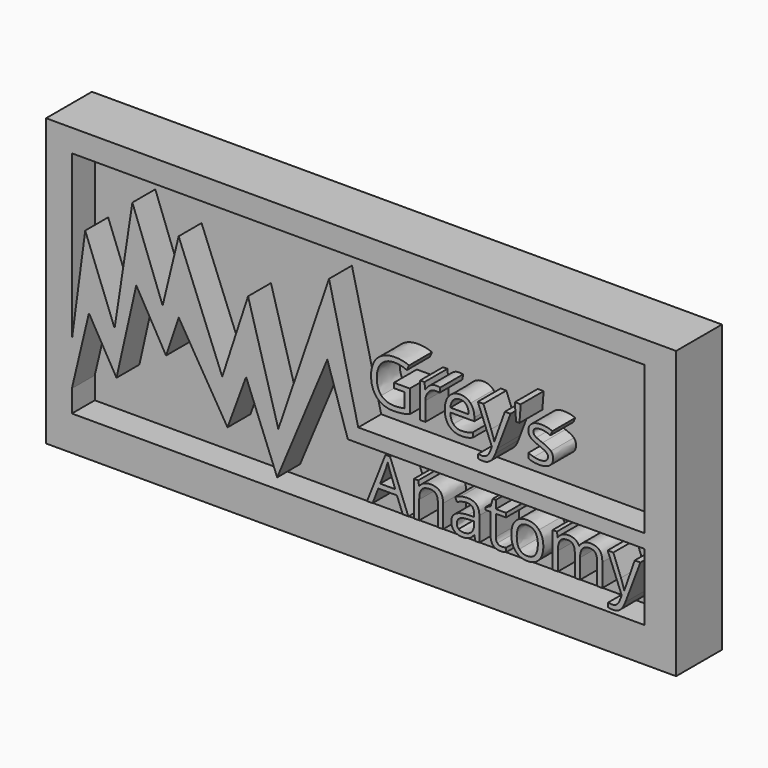
from build123d import *

# Parameters (mm, degrees)
F0_W      = 279.4
F0_H      = 127
F1_DEPTH  = 25.4
F2_DEPTH  = 12.7
F3_DEPTH  = 25.4
F4_DEPTH  = 25.4
F5_DEPTH  = 25.4
F6_DEPTH  = 25.4
F7_DEPTH  = 25.4
F8_DEPTH  = 25.4
F9_DEPTH  = 25.4
F10_DEPTH = 25.4
F11_DEPTH = 25.4
F12_DEPTH = 25.4
F13_DEPTH = 25.4
F14_DEPTH = 25.4
F15_DEPTH = 25.4
F16_DEPTH = 25.4


with BuildPart() as f1:
    # F0 (on Front) → F1 (new body)
    with BuildSketch(Plane.XZ):
        with Locations((-3.9588466167, 0.3931427598)):
            Rectangle(F0_W, F0_H)
        Polygon((-132.2193487672, -18.9143698658), (-132.2193487672, 53.9237214664), (121.7806512328, 53.9237214664), (121.7806512328, 0), (121.7806512328, -11.812004261), (121.7806512328, -17.9444891514), (121.7806512328, -47.6762785336), (-132.2193487672, -47.6762785336), (-132.2193487672, -37.9168875513), align=None, mode=Mode.SUBTRACT)
    extrude(amount=F1_DEPTH)

    # F0 (on Front) → F2 (join)
    with BuildSketch(Plane.XZ):
        Polygon((121.7806512328, 53.9237214664), (-132.2193487672, 53.9237214664), (-132.2193487672, -18.9143698658), (-126.297518611, 25.6726946682), (-113.2765114307, -8.2608237863), (-105.3849980235, 43.4286035597), (-91.969422996, 7.5222076848), (-84.8670601845, 36.9214624689), (-65.5328482389, -11.6113578378), (-54.0901459754, 23.5058874414), (-40.6745709479, -23.958422956), (-18.1837528944, 42.0024342833), (-5.2193487672, -11.812004261), (121.7806512328, -11.812004261), (121.7806512328, 0), align=None)
        with BuildLine():
            Line((24.5695856903, 8.302306513), (24.5695856903, 0))
            Line((24.5695856903, 0), (22.2252456031, 0))
            Line((22.2252456031, 0), (22.2252456031, 15.4708377623))
            Line((22.2252456031, 15.4708377623), (24.1585356943, 15.4708377623))
            Line((24.1585356943, 15.4708377623), (24.4295576697, 12.607038889))
            Line((24.4295576697, 12.607038889), (24.5424834928, 12.607038889))
            add(Edge.make_bspline(
                [(24.5424834928, 12.607038889), (25.4007197482, 14.1157278853), (26.6158016046, 14.9355693609)],
                knots=[0, 0, 0, 1, 1, 1], degree=2))
            add(Edge.make_bspline(
                [(26.6158016046, 14.9355693609), (27.8308834609, 15.7554108365), (29.2853680622, 15.7554108365)],
                knots=[0, 0, 0, 1, 1, 1], degree=2))
            add(Edge.make_bspline(
                [(29.2853680622, 15.7554108365), (30.3152515687, 15.7554108365), (31.1328345279, 15.5837635854)],
                knots=[0, 0, 0, 1, 1, 1], degree=2))
            Line((31.1328345279, 15.5837635854), (30.8076081574, 13.4110707493))
            add(Edge.make_bspline(
                [(30.8076081574, 13.4110707493), (29.8499971776, 13.6233712967), (29.1137208111, 13.6233712967)],
                knots=[0, 0, 0, 1, 1, 1], degree=2))
            add(Edge.make_bspline(
                [(29.1137208111, 13.6233712967), (27.2346351151, 13.6233712967), (25.9021104027, 12.0988726851)],
                knots=[0, 0, 0, 1, 1, 1], degree=2))
            add(Edge.make_bspline(
                [(25.9021104027, 12.0988726851), (24.5695856903, 10.5743740735), (24.5695856903, 8.302306513)],
                knots=[0, 0, 0, 1, 1, 1], degree=2))
        make_face(mode=Mode.SUBTRACT)
        with BuildLine():
            add(Edge.make_bspline(
                [(17.6269060872, 0.7769296628), (16.0347938346, 0.2681554995), (14.391576733, 0)],
                knots=[0, 0, 0, 0.9709878678, 0.9709878678, 0.9709878678], degree=2))
            add(Edge.make_bspline(
                [(14.391576733, 0), (14.3424790734, -0.0080122142), (14.2933357898, -0.0158096152)],
                knots=[0.9709878678, 0.9709878678, 0.9709878678, 1, 1, 1], degree=2))
            add(Edge.make_bspline(
                [(14.2933357898, -0.0158096152), (12.5994484435, -0.2845730742), (10.3680341794, -0.2845730742)],
                knots=[0, 0, 0, 1, 1, 1], degree=2))
            add(Edge.make_bspline(
                [(10.3680341794, -0.2845730742), (8.8718543134, -0.2845730742), (7.5872032589, 0)],
                knots=[0, 0, 0, 0.319412416, 0.319412416, 0.319412416], degree=2))
            add(Edge.make_bspline(
                [(7.5872032589, 0), (4.8499347192, 0.6063537023), (3.0730260083, 2.504694756)],
                knots=[0.319412416, 0.319412416, 0.319412416, 1, 1, 1], degree=2))
            add(Edge.make_bspline(
                [(3.0730260083, 2.504694756), (0.4621809786, 5.2939625861), (0.4621809786, 10.3169031968)],
                knots=[0, 0, 0, 1, 1, 1], degree=2))
            add(Edge.make_bspline(
                [(0.4621809786, 10.3169031968), (0.4621809786, 13.5375476712), (1.7540523947, 15.9586773181)],
                knots=[0, 0, 0, 1, 1, 1], degree=2))
            add(Edge.make_bspline(
                [(1.7540523947, 15.9586773181), (3.0459238107, 18.3798069649), (5.473829007, 19.6558687658)],
                knots=[0, 0, 0, 1, 1, 1], degree=2))
            add(Edge.make_bspline(
                [(5.473829007, 19.6558687658), (7.9017342033, 20.9319305666), (11.158514941, 20.9319305666)],
                knots=[0, 0, 0, 1, 1, 1], degree=2))
            add(Edge.make_bspline(
                [(11.158514941, 20.9319305666), (14.4649830409, 20.9319305666), (17.3152308155, 19.7213657432)],
                knots=[0, 0, 0, 1, 1, 1], degree=2))
            Line((17.3152308155, 19.7213657432), (16.3847220333, 17.6028773021))
            add(Edge.make_bspline(
                [(16.3847220333, 17.6028773021), (13.5886786537, 18.786339928), (11.0049358216, 18.786339928)],
                knots=[0, 0, 0, 1, 1, 1], degree=2))
            add(Edge.make_bspline(
                [(11.0049358216, 18.786339928), (7.2377303636, 18.786339928), (5.1192419225, 16.5436330816)],
                knots=[0, 0, 0, 1, 1, 1], degree=2))
            add(Edge.make_bspline(
                [(5.1192419225, 16.5436330816), (3.0007534815, 14.3009262352), (3.0007534815, 10.3169031968)],
                knots=[0, 0, 0, 1, 1, 1], degree=2))
            add(Edge.make_bspline(
                [(3.0007534815, 10.3169031968), (3.0007534815, 6.1386477428), (5.0401938464, 3.9795060054)],
                knots=[0, 0, 0, 1, 1, 1], degree=2))
            add(Edge.make_bspline(
                [(5.0401938464, 3.9795060054), (7.0796342112, 1.8203642681), (11.0320380191, 1.8203642681)],
                knots=[0, 0, 0, 1, 1, 1], degree=2))
            add(Edge.make_bspline(
                [(11.0320380191, 1.8203642681), (13.1776286577, 1.8203642681), (15.223844572, 2.3172378897)],
                knots=[0, 0, 0, 1, 1, 1], degree=2))
            Line((15.223844572, 2.3172378897), (15.223844572, 8.6681861798))
            Line((15.223844572, 8.6681861798), (10.6119539573, 8.6681861798))
            Line((10.6119539573, 8.6681861798), (10.6119539573, 10.8137768184))
            Line((10.6119539573, 10.8137768184), (17.6269060872, 10.8137768184))
            Line((17.6269060872, 10.8137768184), (17.6269060872, 0.7769296628))
        make_face(mode=Mode.SUBTRACT)
        with BuildLine():
            add(Edge.make_bspline(
                [(45.5873398825, 0.7182082348), (44.4687381201, 0.2382263877), (43.4600252029, 0)],
                knots=[0, 0, 0, 0.9005120931, 0.9005120931, 0.9005120931], degree=2))
            add(Edge.make_bspline(
                [(43.4600252029, 0), (43.3485833493, -0.0263190743), (43.2384827623, -0.0496873622)],
                knots=[0.9005120931, 0.9005120931, 0.9005120931, 1, 1, 1], degree=2))
            add(Edge.make_bspline(
                [(43.2384827623, -0.0496873622), (42.1318096961, -0.2845730742), (40.5643992717, -0.2845730742)],
                knots=[0, 0, 0, 1, 1, 1], degree=2))
            add(Edge.make_bspline(
                [(40.5643992717, -0.2845730742), (39.2997362762, -0.2845730742), (38.2314471408, 0)],
                knots=[0, 0, 0, 0.3688754729, 0.3688754729, 0.3688754729], degree=2))
            add(Edge.make_bspline(
                [(38.2314471408, 0), (36.4036664259, 0.4868880153), (35.1507353132, 1.8068131693)],
                knots=[0.3688754729, 0.3688754729, 0.3688754729, 1, 1, 1], degree=2))
            add(Edge.make_bspline(
                [(35.1507353132, 1.8068131693), (33.1654993434, 3.8981994128), (33.1654993434, 7.6066834429)],
                knots=[0, 0, 0, 1, 1, 1], degree=2))
            add(Edge.make_bspline(
                [(33.1654993434, 7.6066834429), (33.1654993434, 11.3513037363), (35.0084487761, 13.5533572864)],
                knots=[0, 0, 0, 1, 1, 1], degree=2))
            add(Edge.make_bspline(
                [(35.0084487761, 13.5533572864), (36.8513982088, 15.7554108365), (39.95911686, 15.7554108365)],
                knots=[0, 0, 0, 1, 1, 1], degree=2))
            add(Edge.make_bspline(
                [(39.95911686, 15.7554108365), (42.8635690297, 15.7554108365), (44.5574563759, 13.8424473935)],
                knots=[0, 0, 0, 1, 1, 1], degree=2))
            add(Edge.make_bspline(
                [(44.5574563759, 13.8424473935), (46.2513437222, 11.9294839505), (46.2513437222, 8.7946631017)],
                knots=[0, 0, 0, 1, 1, 1], degree=2))
            Line((46.2513437222, 8.7946631017), (46.2513437222, 7.3130763028))
            Line((46.2513437222, 7.3130763028), (35.5956630561, 7.3130763028))
            add(Edge.make_bspline(
                [(35.5956630561, 7.3130763028), (35.6679355829, 4.5893054501), (36.9733580977, 3.1777326615)],
                knots=[0, 0, 0, 1, 1, 1], degree=2))
            add(Edge.make_bspline(
                [(36.9733580977, 3.1777326615), (38.2787806125, 1.766159873), (40.6502228973, 1.766159873)],
                knots=[0, 0, 0, 1, 1, 1], degree=2))
            add(Edge.make_bspline(
                [(40.6502228973, 1.766159873), (43.1481421039, 1.766159873), (45.5873398825, 2.8095944783)],
                knots=[0, 0, 0, 1, 1, 1], degree=2))
            Line((45.5873398825, 2.8095944783), (45.5873398825, 0.7182082348))
        make_face(mode=Mode.SUBTRACT)
        with BuildLine():
            Line((62.3048787316, 15.4708377623), (56.4656291967, 0))
            Line((56.4656291967, 0), (55.6558062685, -2.1455906386))
            add(Edge.make_bspline(
                [(55.6558062685, -2.1455906386), (54.6665760583, -4.7564356682), (53.3476024447, -5.8518161521)],
                knots=[0, 0, 0, 1, 1, 1], degree=2))
            add(Edge.make_bspline(
                [(53.3476024447, -5.8518161521), (52.0286288311, -6.947196636), (50.1088898387, -6.947196636)],
                knots=[0, 0, 0, 1, 1, 1], degree=2))
            add(Edge.make_bspline(
                [(50.1088898387, -6.947196636), (49.0338360029, -6.947196636), (47.9904013977, -6.7032768582)],
                knots=[0, 0, 0, 1, 1, 1], degree=2))
            Line((47.9904013977, -6.7032768582), (47.9904013977, -4.828708195))
            add(Edge.make_bspline(
                [(47.9904013977, -4.828708195), (48.7673310605, -4.9958384132), (49.7249420402, -4.9958384132)],
                knots=[0, 0, 0, 1, 1, 1], degree=2))
            add(Edge.make_bspline(
                [(49.7249420402, -4.9958384132), (52.1415546542, -4.9958384132), (53.1714381607, -2.2856186592)],
                knots=[0, 0, 0, 1, 1, 1], degree=2))
            Line((53.1714381607, -2.2856186592), (54.034191449, -0.0858236255))
            Line((54.034191449, -0.0858236255), (53.9997523519, 0))
            Line((53.9997523519, 0), (47.791651949, 15.4708377623))
            Line((47.791651949, 15.4708377623), (50.3076392873, 15.4708377623))
            Line((50.3076392873, 15.4708377623), (53.6954139798, 6.6490724631))
            add(Edge.make_bspline(
                [(53.6954139798, 6.6490724631), (54.8066040789, 3.6271774374), (55.0776260543, 2.2856186592)],
                knots=[0, 0, 0, 1, 1, 1], degree=2))
            Line((55.0776260543, 2.2856186592), (55.1905518774, 2.2856186592))
            add(Edge.make_bspline(
                [(55.1905518774, 2.2856186592), (55.3712331943, 3.0083439269), (55.9584474744, 4.7519186353)],
                knots=[0, 0, 0, 1, 1, 1], degree=2))
            add(Edge.make_bspline(
                [(55.9584474744, 4.7519186353), (56.5456617544, 6.4954933437), (59.7934084263, 15.4708377623)],
                knots=[0, 0, 0, 1, 1, 1], degree=2))
            Line((59.7934084263, 15.4708377623), (62.3048787316, 15.4708377623))
        make_face(mode=Mode.SUBTRACT)
        Polygon((64.2110666253, 20.6383234266), (66.8354627537, 20.6383234266), (66.2708336383, 13.1852191031), (64.7892468394, 13.1852191031), align=None, mode=Mode.SUBTRACT)
        with BuildLine():
            add(Edge.make_bspline(
                [(79.5825296633, 0.8875969694), (78.7667936579, 0.2929804149), (77.6162938443, 0)],
                knots=[0, 0, 0, 0.5072784088, 0.5072784088, 0.5072784088], degree=2))
            add(Edge.make_bspline(
                [(77.6162938443, 0), (76.4988086744, -0.2845730742), (75.06549674, -0.2845730742)],
                knots=[0.5072784088, 0.5072784088, 0.5072784088, 1, 1, 1], degree=2))
            add(Edge.make_bspline(
                [(75.06549674, -0.2845730742), (73.4042131809, -0.2845730742), (72.1381700027, 0)],
                knots=[0, 0, 0, 0.5400617249, 0.5400617249, 0.5400617249], degree=2))
            add(Edge.make_bspline(
                [(72.1381700027, 0), (71.0599567377, 0.2423538697), (70.2684077754, 0.6911060373)],
                knots=[0.5400617249, 0.5400617249, 0.5400617249, 1, 1, 1], degree=2))
            Line((70.2684077754, 0.6911060373), (70.2684077754, 2.8637988734))
            add(Edge.make_bspline(
                [(70.2684077754, 2.8637988734), (71.3841149075, 2.299169758), (72.6601767083, 1.9762019039)],
                knots=[0, 0, 0, 1, 1, 1], degree=2))
            add(Edge.make_bspline(
                [(72.6601767083, 1.9762019039), (73.9362385091, 1.6532340499), (75.124218168, 1.6532340499)],
                knots=[0, 0, 0, 1, 1, 1], degree=2))
            add(Edge.make_bspline(
                [(75.124218168, 1.6532340499), (76.9581335348, 1.6532340499), (77.9451052286, 2.2381898135)],
                knots=[0, 0, 0, 1, 1, 1], degree=2))
            add(Edge.make_bspline(
                [(77.9451052286, 2.2381898135), (78.9320769223, 2.8231455771), (78.9320769223, 4.0246763347)],
                knots=[0, 0, 0, 1, 1, 1], degree=2))
            add(Edge.make_bspline(
                [(78.9320769223, 4.0246763347), (78.9320769223, 4.9280829193), (78.1506302266, 5.5695015944)],
                knots=[0, 0, 0, 1, 1, 1], degree=2))
            add(Edge.make_bspline(
                [(78.1506302266, 5.5695015944), (77.3691835309, 6.2109202696), (75.0925989375, 7.0872246567)],
                knots=[0, 0, 0, 1, 1, 1], degree=2))
            add(Edge.make_bspline(
                [(75.0925989375, 7.0872246567), (72.9334572002, 7.891256517), (72.0232750661, 8.4920218958)],
                knots=[0, 0, 0, 1, 1, 1], degree=2))
            add(Edge.make_bspline(
                [(72.0232750661, 8.4920218958), (71.1130929321, 9.0927872746), (70.6681651891, 9.8539073222)],
                knots=[0, 0, 0, 1, 1, 1], degree=2))
            add(Edge.make_bspline(
                [(70.6681651891, 9.8539073222), (70.2232374462, 10.6150273698), (70.2232374462, 11.6720130738)],
                knots=[0, 0, 0, 1, 1, 1], degree=2))
            add(Edge.make_bspline(
                [(70.2232374462, 11.6720130738), (70.2232374462, 13.5646498687), (71.763545673, 14.6600303526)],
                knots=[0, 0, 0, 1, 1, 1], degree=2))
            add(Edge.make_bspline(
                [(71.763545673, 14.6600303526), (73.3038538999, 15.7554108365), (75.9824544234, 15.7554108365)],
                knots=[0, 0, 0, 1, 1, 1], degree=2))
            add(Edge.make_bspline(
                [(75.9824544234, 15.7554108365), (78.48037363, 15.7554108365), (80.8698840464, 14.7390784288)],
                knots=[0, 0, 0, 1, 1, 1], degree=2))
            Line((80.8698840464, 14.7390784288), (80.0342329556, 12.8328905351))
            add(Edge.make_bspline(
                [(80.0342329556, 12.8328905351), (77.7079610001, 13.7905015149), (75.8153242052, 13.7905015149)],
                knots=[0, 0, 0, 1, 1, 1], degree=2))
            add(Edge.make_bspline(
                [(75.8153242052, 13.7905015149), (74.1485390565, 13.7905015149), (73.3015953834, 13.2687842122)],
                knots=[0, 0, 0, 1, 1, 1], degree=2))
            add(Edge.make_bspline(
                [(73.3015953834, 13.2687842122), (72.4546517103, 12.7470669096), (72.4546517103, 11.8301092261)],
                knots=[0, 0, 0, 1, 1, 1], degree=2))
            add(Edge.make_bspline(
                [(72.4546517103, 11.8301092261), (72.4546517103, 11.2067586827), (72.7731025314, 10.7708650056)],
                knots=[0, 0, 0, 1, 1, 1], degree=2))
            add(Edge.make_bspline(
                [(72.7731025314, 10.7708650056), (73.0915533525, 10.3349713285), (73.7962104885, 9.9397309477)],
                knots=[0, 0, 0, 1, 1, 1], degree=2))
            add(Edge.make_bspline(
                [(73.7962104885, 9.9397309477), (74.5008676246, 9.544490567), (76.5064302425, 8.7946631017)],
                knots=[0, 0, 0, 1, 1, 1], degree=2))
            add(Edge.make_bspline(
                [(76.5064302425, 8.7946631017), (79.2573032928, 7.7918817927), (80.2239483384, 6.775549385)],
                knots=[0, 0, 0, 1, 1, 1], degree=2))
            add(Edge.make_bspline(
                [(80.2239483384, 6.775549385), (81.190593384, 5.7592169772), (81.190593384, 4.2189087504)],
                knots=[0, 0, 0, 1, 1, 1], degree=2))
            add(Edge.make_bspline(
                [(81.190593384, 4.2189087504), (81.190593384, 2.059767013), (79.5825296633, 0.8875969694)],
                knots=[0, 0, 0, 1, 1, 1], degree=2))
        make_face(mode=Mode.SUBTRACT)
        Polygon((-124.6507890017, -6.0345723474), (-132.2193487672, -37.9168875513), (-132.2193487672, -47.6762785336), (121.7806512328, -47.6762785336), (121.7806512328, -17.9444891514), (-9.844164013, -17.9444891514), (-18.9298406458, 10.2524342833), (-41.1740798718, -43.008422956), (-54.9592409498, -8.2322154307), (-63.1971969822, -30.6613578378), (-84.8148405174, 5.1714624689), (-90.4542222241, -11.4674386158), (-103.6597467454, 11.6786035597), (-112.4321199448, -27.3108237863), align=None)
        with BuildLine():
            Line((32.4066378122, -39.3162545645), (30.062297725, -39.3162545645))
            Line((30.062297725, -39.3162545645), (30.062297725, -29.3065096064))
            add(Edge.make_bspline(
                [(30.062297725, -29.3065096064), (30.062297725, -27.4183898445), (29.2018029532, -26.4856225458)],
                knots=[0, 0, 0, 1, 1, 1], degree=2))
            add(Edge.make_bspline(
                [(29.2018029532, -26.4856225458), (28.3413081813, -25.5528552472), (26.5028757815, -25.5528552472)],
                knots=[0, 0, 0, 1, 1, 1], degree=2))
            add(Edge.make_bspline(
                [(26.5028757815, -25.5528552472), (24.0772291017, -25.5528552472), (22.9479708708, -26.8650533114)],
                knots=[0, 0, 0, 1, 1, 1], degree=2))
            add(Edge.make_bspline(
                [(22.9479708708, -26.8650533114), (21.81871264, -28.1772513756), (21.81871264, -31.1991464013)],
                knots=[0, 0, 0, 1, 1, 1], degree=2))
            Line((21.81871264, -31.1991464013), (21.81871264, -39.3162545645))
            Line((21.81871264, -39.3162545645), (19.4743725528, -39.3162545645))
            Line((19.4743725528, -39.3162545645), (19.4743725528, -23.8454168021))
            Line((19.4743725528, -23.8454168021), (21.3805604464, -23.8454168021))
            Line((21.3805604464, -23.8454168021), (21.759991212, -25.9639052432))
            Line((21.759991212, -25.9639052432), (21.8729170351, -25.9639052432))
            add(Edge.make_bspline(
                [(21.8729170351, -25.9639052432), (22.5956423028, -24.8210959136), (23.8942892683, -24.1909698208)],
                knots=[0, 0, 0, 1, 1, 1], degree=2))
            add(Edge.make_bspline(
                [(23.8942892683, -24.1909698208), (25.1929362337, -23.560843728), (26.7874488556, -23.560843728)],
                knots=[0, 0, 0, 1, 1, 1], degree=2))
            add(Edge.make_bspline(
                [(26.7874488556, -23.560843728), (29.5834922352, -23.560843728), (30.9950650237, -24.9091780556)],
                knots=[0, 0, 0, 1, 1, 1], degree=2))
            add(Edge.make_bspline(
                [(30.9950650237, -24.9091780556), (32.4066378122, -26.2575123832), (32.4066378122, -29.2252030138)],
                knots=[0, 0, 0, 1, 1, 1], degree=2))
            Line((32.4066378122, -29.2252030138), (32.4066378122, -39.3162545645))
        make_face(mode=Mode.SUBTRACT)
        with BuildLine():
            Line((48.4692068875, -39.3162545645), (46.7301492121, -39.3162545645))
            Line((46.7301492121, -39.3162545645), (46.264894821, -37.1119424979))
            Line((46.264894821, -37.1119424979), (46.1519689979, -37.1119424979))
            add(Edge.make_bspline(
                [(46.1519689979, -37.1119424979), (44.9956085695, -38.5664270992), (43.8460236905, -39.0836273689)],
                knots=[0, 0, 0, 1, 1, 1], degree=2))
            add(Edge.make_bspline(
                [(43.8460236905, -39.0836273689), (42.6964388115, -39.6008276387), (40.9709322348, -39.6008276387)],
                knots=[0, 0, 0, 1, 1, 1], degree=2))
            add(Edge.make_bspline(
                [(40.9709322348, -39.6008276387), (38.6717624769, -39.6008276387), (37.366339962, -38.4128479798)],
                knots=[0, 0, 0, 1, 1, 1], degree=2))
            add(Edge.make_bspline(
                [(37.366339962, -38.4128479798), (36.0609174472, -37.224868321), (36.0609174472, -35.0386243861)],
                knots=[0, 0, 0, 1, 1, 1], degree=2))
            add(Edge.make_bspline(
                [(36.0609174472, -35.0386243861), (36.0609174472, -30.3544612446), (43.554675067, -30.1286095985)],
                knots=[0, 0, 0, 1, 1, 1], degree=2))
            Line((43.554675067, -30.1286095985), (46.1790711954, -30.0427859729))
            Line((46.1790711954, -30.0427859729), (46.1790711954, -29.0806579603))
            add(Edge.make_bspline(
                [(46.1790711954, -29.0806579603), (46.1790711954, -27.2602936922), (45.3976244997, -26.3930233709)],
                knots=[0, 0, 0, 1, 1, 1], degree=2))
            add(Edge.make_bspline(
                [(45.3976244997, -26.3930233709), (44.6161778039, -25.5257530496), (42.8906712272, -25.5257530496)],
                knots=[0, 0, 0, 1, 1, 1], degree=2))
            add(Edge.make_bspline(
                [(42.8906712272, -25.5257530496), (40.9573811361, -25.5257530496), (38.5181833575, -26.7092156755)],
                knots=[0, 0, 0, 1, 1, 1], degree=2))
            Line((38.5181833575, -26.7092156755), (37.7954580897, -24.915953605))
            add(Edge.make_bspline(
                [(37.7954580897, -24.915953605), (38.9382674193, -24.2971200945), (40.3001528457, -23.9447915265)],
                knots=[0, 0, 0, 1, 1, 1], degree=2))
            add(Edge.make_bspline(
                [(40.3001528457, -23.9447915265), (41.6620382721, -23.5924629584), (43.0352162808, -23.5924629584)],
                knots=[0, 0, 0, 1, 1, 1], degree=2))
            add(Edge.make_bspline(
                [(43.0352162808, -23.5924629584), (45.7996404299, -23.5924629584), (47.1344236587, -24.8188373971)],
                knots=[0, 0, 0, 1, 1, 1], degree=2))
            add(Edge.make_bspline(
                [(47.1344236587, -24.8188373971), (48.4692068875, -26.0452118358), (48.4692068875, -28.7554315898)],
                knots=[0, 0, 0, 1, 1, 1], degree=2))
            Line((48.4692068875, -28.7554315898), (48.4692068875, -39.3162545645))
        make_face(mode=Mode.SUBTRACT)
        with BuildLine():
            add(Edge.make_bspline(
                [(74.9367613017, -25.7222439818), (76.8497247447, -27.8836442356), (76.8497247447, -31.5650260681)],
                knots=[0, 0, 0, 1, 1, 1], degree=2))
            add(Edge.make_bspline(
                [(76.8497247447, -31.5650260681), (76.8497247447, -35.3502996578), (74.9457953675, -37.4755636482)],
                knots=[0, 0, 0, 1, 1, 1], degree=2))
            add(Edge.make_bspline(
                [(74.9457953675, -37.4755636482), (73.0418659903, -39.6008276387), (69.6811934954, -39.6008276387)],
                knots=[0, 0, 0, 1, 1, 1], degree=2))
            add(Edge.make_bspline(
                [(69.6811934954, -39.6008276387), (67.6033583507, -39.6008276387), (65.99529463, -38.6251485272)],
                knots=[0, 0, 0, 1, 1, 1], degree=2))
            add(Edge.make_bspline(
                [(65.99529463, -38.6251485272), (64.3872309093, -37.6494694158), (63.5109265221, -35.8291051477)],
                knots=[0, 0, 0, 1, 1, 1], degree=2))
            add(Edge.make_bspline(
                [(63.5109265221, -35.8291051477), (62.634622135, -34.0087408796), (62.634622135, -31.5650260681)],
                knots=[0, 0, 0, 1, 1, 1], degree=2))
            add(Edge.make_bspline(
                [(62.634622135, -31.5650260681), (62.634622135, -27.7842695113), (64.5272589299, -25.6725566196)],
                knots=[0, 0, 0, 1, 1, 1], degree=2))
            add(Edge.make_bspline(
                [(64.5272589299, -25.6725566196), (66.4198957248, -23.560843728), (69.7805682197, -23.560843728)],
                knots=[0, 0, 0, 1, 1, 1], degree=2))
            add(Edge.make_bspline(
                [(69.7805682197, -23.560843728), (73.0237978586, -23.560843728), (74.9367613017, -25.7222439818)],
                knots=[0, 0, 0, 1, 1, 1], degree=2))
        make_face(mode=Mode.SUBTRACT)
        with BuildLine():
            Line((103.0214135023, -39.3162545645), (100.6815904481, -39.3162545645))
            Line((100.6815904481, -39.3162545645), (100.6815904481, -29.2523052114))
            add(Edge.make_bspline(
                [(100.6815904481, -29.2523052114), (100.6815904481, -27.4003217128), (99.8911096865, -26.47658848)],
                knots=[0, 0, 0, 1, 1, 1], degree=2))
            add(Edge.make_bspline(
                [(99.8911096865, -26.47658848), (99.1006289249, -25.5528552472), (97.4338437762, -25.5528552472)],
                knots=[0, 0, 0, 1, 1, 1], degree=2))
            add(Edge.make_bspline(
                [(97.4338437762, -25.5528552472), (95.2475998413, -25.5528552472), (94.2019067196, -26.8085903998)],
                knots=[0, 0, 0, 1, 1, 1], degree=2))
            add(Edge.make_bspline(
                [(94.2019067196, -26.8085903998), (93.1562135978, -28.0643255525), (93.1562135978, -30.6751705822)],
                knots=[0, 0, 0, 1, 1, 1], degree=2))
            Line((93.1562135978, -30.6751705822), (93.1562135978, -39.3162545645))
            Line((93.1562135978, -39.3162545645), (90.8118735106, -39.3162545645))
            Line((90.8118735106, -39.3162545645), (90.8118735106, -29.2523052114))
            add(Edge.make_bspline(
                [(90.8118735106, -29.2523052114), (90.8118735106, -27.4003217128), (90.0213927491, -26.47658848)],
                knots=[0, 0, 0, 1, 1, 1], degree=2))
            add(Edge.make_bspline(
                [(90.0213927491, -26.47658848), (89.2309119875, -25.5528552472), (87.55057574, -25.5528552472)],
                knots=[0, 0, 0, 1, 1, 1], degree=2))
            add(Edge.make_bspline(
                [(87.55057574, -25.5528552472), (85.3507807063, -25.5528552472), (84.3276727492, -26.8718288608)],
                knots=[0, 0, 0, 1, 1, 1], degree=2))
            add(Edge.make_bspline(
                [(84.3276727492, -26.8718288608), (83.3045647921, -28.1908024744), (83.3045647921, -31.1991464013)],
                knots=[0, 0, 0, 1, 1, 1], degree=2))
            Line((83.3045647921, -31.1991464013), (83.3045647921, -39.3162545645))
            Line((83.3045647921, -39.3162545645), (80.9602247049, -39.3162545645))
            Line((80.9602247049, -39.3162545645), (80.9602247049, -23.8454168021))
            Line((80.9602247049, -23.8454168021), (82.8664125985, -23.8454168021))
            Line((82.8664125985, -23.8454168021), (83.2458433641, -25.9639052432))
            Line((83.2458433641, -25.9639052432), (83.3587691872, -25.9639052432))
            add(Edge.make_bspline(
                [(83.3587691872, -25.9639052432), (84.0227730269, -24.8346470124), (85.2310793339, -24.1977453702)],
                knots=[0, 0, 0, 1, 1, 1], degree=2))
            add(Edge.make_bspline(
                [(85.2310793339, -24.1977453702), (86.4393856409, -23.560843728), (87.9345235385, -23.560843728)],
                knots=[0, 0, 0, 1, 1, 1], degree=2))
            add(Edge.make_bspline(
                [(87.9345235385, -23.560843728), (91.5617009759, -23.560843728), (92.677408108, -26.1897568893)],
                knots=[0, 0, 0, 1, 1, 1], degree=2))
            Line((92.677408108, -26.1897568893), (92.790333931, -26.1897568893))
            add(Edge.make_bspline(
                [(92.790333931, -26.1897568893), (93.4814399683, -24.974675033), (94.7936380325, -24.2677593805)],
                knots=[0, 0, 0, 1, 1, 1], degree=2))
            add(Edge.make_bspline(
                [(94.7936380325, -24.2677593805), (96.1058360967, -23.560843728), (97.7861723442, -23.560843728)],
                knots=[0, 0, 0, 1, 1, 1], degree=2))
            add(Edge.make_bspline(
                [(97.7861723442, -23.560843728), (100.4105684727, -23.560843728), (101.7159909875, -24.9091780556)],
                knots=[0, 0, 0, 1, 1, 1], degree=2))
            add(Edge.make_bspline(
                [(101.7159909875, -24.9091780556), (103.0214135023, -26.2575123832), (103.0214135023, -29.2252030138)],
                knots=[0, 0, 0, 1, 1, 1], degree=2))
            Line((103.0214135023, -29.2252030138), (103.0214135023, -39.3162545645))
        make_face(mode=Mode.SUBTRACT)
        with BuildLine():
            Line((111.6353952871, -39.40207819), (105.3928557871, -23.8454168021))
            Line((105.3928557871, -23.8454168021), (107.9088431254, -23.8454168021))
            Line((107.9088431254, -23.8454168021), (111.2966178178, -32.6671821014))
            add(Edge.make_bspline(
                [(111.2966178178, -32.6671821014), (112.407807917, -35.6890771271), (112.6788298924, -37.0306359053)],
                knots=[0, 0, 0, 1, 1, 1], degree=2))
            Line((112.6788298924, -37.0306359053), (112.7917557155, -37.0306359053))
            add(Edge.make_bspline(
                [(112.7917557155, -37.0306359053), (112.9724370324, -36.3079106376), (113.5596513124, -34.5643359292)],
                knots=[0, 0, 0, 1, 1, 1], degree=2))
            add(Edge.make_bspline(
                [(113.5596513124, -34.5643359292), (114.1468655924, -32.8207612208), (117.3946122643, -23.8454168021)],
                knots=[0, 0, 0, 1, 1, 1], degree=2))
            Line((117.3946122643, -23.8454168021), (119.9060825697, -23.8454168021))
            Line((119.9060825697, -23.8454168021), (113.2570101066, -41.4618452031))
            add(Edge.make_bspline(
                [(113.2570101066, -41.4618452031), (112.2677798963, -44.0726902327), (110.9488062827, -45.1680707166)],
                knots=[0, 0, 0, 1, 1, 1], degree=2))
            add(Edge.make_bspline(
                [(110.9488062827, -45.1680707166), (109.6298326691, -46.2634512005), (107.7100936767, -46.2634512005)],
                knots=[0, 0, 0, 1, 1, 1], degree=2))
            add(Edge.make_bspline(
                [(107.7100936767, -46.2634512005), (106.635039841, -46.2634512005), (105.5916052357, -46.0195314227)],
                knots=[0, 0, 0, 1, 1, 1], degree=2))
            Line((105.5916052357, -46.0195314227), (105.5916052357, -44.1449627595))
            add(Edge.make_bspline(
                [(105.5916052357, -44.1449627595), (106.3685348985, -44.3120929777), (107.3261458782, -44.3120929777)],
                knots=[0, 0, 0, 1, 1, 1], degree=2))
            add(Edge.make_bspline(
                [(107.3261458782, -44.3120929777), (109.7427584922, -44.3120929777), (110.7726419987, -41.6018732237)],
                knots=[0, 0, 0, 1, 1, 1], degree=2))
            Line((110.7726419987, -41.6018732237), (111.6353952871, -39.40207819))
        make_face(mode=Mode.SUBTRACT)
        Polygon((16.990004445, -39.3162545645), (14.5056363372, -39.3162545645), (11.9354446038, -32.7530057269), (3.6647573212, -32.7530057269), (1.1261848183, -39.3162545645), (-1.3039788944, -39.3162545645), (6.8537825651, -18.5921075123), (8.8728962818, -18.5921075123), align=None, mode=Mode.SUBTRACT)
        with BuildLine():
            add(Edge.make_bspline(
                [(56.4688721947, -36.9154515657), (57.1328760344, -37.6630205146), (58.2892364628, -37.6630205146)],
                knots=[0, 0, 0, 1, 1, 1], degree=2))
            add(Edge.make_bspline(
                [(58.2892364628, -37.6630205146), (58.9125870062, -37.6630205146), (59.4907672204, -37.5726798561)],
                knots=[0, 0, 0, 1, 1, 1], degree=2))
            add(Edge.make_bspline(
                [(59.4907672204, -37.5726798561), (60.0689474346, -37.4823391976), (60.4077249038, -37.3829644733)],
                knots=[0, 0, 0, 1, 1, 1], degree=2))
            Line((60.4077249038, -37.3829644733), (60.4077249038, -39.1762265439))
            add(Edge.make_bspline(
                [(60.4077249038, -39.1762265439), (60.0282941383, -39.3569078608), (59.2875007389, -39.4788677497)],
                knots=[0, 0, 0, 1, 1, 1], degree=2))
            add(Edge.make_bspline(
                [(59.2875007389, -39.4788677497), (58.5467073394, -39.6008276387), (57.9504589936, -39.6008276387)],
                knots=[0, 0, 0, 1, 1, 1], degree=2))
            add(Edge.make_bspline(
                [(57.9504589936, -39.6008276387), (53.4650453007, -39.6008276387), (53.4650453007, -34.8714941679)],
                knots=[0, 0, 0, 1, 1, 1], degree=2))
            Line((53.4650453007, -34.8714941679), (53.4650453007, -25.6657810702))
            Line((53.4650453007, -25.6657810702), (51.2471821354, -25.6657810702))
            Line((51.2471821354, -25.6657810702), (51.2471821354, -24.5365228394))
            Line((51.2471821354, -24.5365228394), (53.4650453007, -23.560843728))
            Line((53.4650453007, -23.560843728), (54.449758478, -20.258892661))
            Line((54.449758478, -20.258892661), (55.804868355, -20.258892661))
            Line((55.804868355, -20.258892661), (55.804868355, -23.8454168021))
            Line((55.804868355, -23.8454168021), (60.2947990808, -23.8454168021))
            Line((60.2947990808, -23.8454168021), (60.2947990808, -25.6657810702))
            Line((60.2947990808, -25.6657810702), (55.804868355, -25.6657810702))
            Line((55.804868355, -25.6657810702), (55.804868355, -34.7721194436))
            add(Edge.make_bspline(
                [(55.804868355, -34.7721194436), (55.804868355, -36.1678826169), (56.4688721947, -36.9154515657)],
                knots=[0, 0, 0, 1, 1, 1], degree=2))
        make_face(mode=Mode.SUBTRACT)
    extrude(amount=F2_DEPTH)

    # F0 (on Front) → F3 (join)
    with BuildSketch(Plane.XZ):
        Polygon((-126.297518611, 25.6726946682), (-132.2193487672, -18.9143698658), (-132.2193487672, -37.9168875513), (-124.6507890017, -6.0345723474), (-112.4321199448, -27.3108237863), (-103.6597467454, 11.6786035597), (-90.4542222241, -11.4674386158), (-84.8148405174, 5.1714624689), (-63.1971969822, -30.6613578378), (-54.9592409498, -8.2322154307), (-41.1740798718, -43.008422956), (-18.9298406458, 10.2524342833), (-9.844164013, -17.9444891514), (121.7806512328, -17.9444891514), (121.7806512328, -11.812004261), (-5.2193487672, -11.812004261), (-18.1837528944, 42.0024342833), (-40.6745709479, -23.958422956), (-54.0901459754, 23.5058874414), (-65.5328482389, -11.6113578378), (-84.8670601845, 36.9214624689), (-91.969422996, 7.5222076848), (-105.3849980235, 43.4286035597), (-113.2765114307, -8.2608237863), align=None)
    extrude(amount=F3_DEPTH)

    # F0 (on Front) → F4 (join)
    with BuildSketch(Plane.XZ):
        with BuildLine():
            Line((7.5872032589, 0), (14.391576733, 0))
            add(Edge.make_bspline(
                [(17.6269060872, 0.7769296628), (16.0347938346, 0.2681554995), (14.391576733, 0)],
                knots=[0, 0, 0, 0.9709878678, 0.9709878678, 0.9709878678], degree=2))
            Line((17.6269060872, 0.7769296628), (17.6269060872, 10.8137768184))
            Line((17.6269060872, 10.8137768184), (10.6119539573, 10.8137768184))
            Line((10.6119539573, 10.8137768184), (10.6119539573, 8.6681861798))
            Line((10.6119539573, 8.6681861798), (15.223844572, 8.6681861798))
            Line((15.223844572, 8.6681861798), (15.223844572, 2.3172378897))
            add(Edge.make_bspline(
                [(11.0320380191, 1.8203642681), (13.1776286577, 1.8203642681), (15.223844572, 2.3172378897)],
                knots=[0, 0, 0, 1, 1, 1], degree=2))
            add(Edge.make_bspline(
                [(5.0401938464, 3.9795060054), (7.0796342112, 1.8203642681), (11.0320380191, 1.8203642681)],
                knots=[0, 0, 0, 1, 1, 1], degree=2))
            add(Edge.make_bspline(
                [(3.0007534815, 10.3169031968), (3.0007534815, 6.1386477428), (5.0401938464, 3.9795060054)],
                knots=[0, 0, 0, 1, 1, 1], degree=2))
            add(Edge.make_bspline(
                [(5.1192419225, 16.5436330816), (3.0007534815, 14.3009262352), (3.0007534815, 10.3169031968)],
                knots=[0, 0, 0, 1, 1, 1], degree=2))
            add(Edge.make_bspline(
                [(11.0049358216, 18.786339928), (7.2377303636, 18.786339928), (5.1192419225, 16.5436330816)],
                knots=[0, 0, 0, 1, 1, 1], degree=2))
            add(Edge.make_bspline(
                [(16.3847220333, 17.6028773021), (13.5886786537, 18.786339928), (11.0049358216, 18.786339928)],
                knots=[0, 0, 0, 1, 1, 1], degree=2))
            Line((16.3847220333, 17.6028773021), (17.3152308155, 19.7213657432))
            add(Edge.make_bspline(
                [(11.158514941, 20.9319305666), (14.4649830409, 20.9319305666), (17.3152308155, 19.7213657432)],
                knots=[0, 0, 0, 1, 1, 1], degree=2))
            add(Edge.make_bspline(
                [(5.473829007, 19.6558687658), (7.9017342033, 20.9319305666), (11.158514941, 20.9319305666)],
                knots=[0, 0, 0, 1, 1, 1], degree=2))
            add(Edge.make_bspline(
                [(1.7540523947, 15.9586773181), (3.0459238107, 18.3798069649), (5.473829007, 19.6558687658)],
                knots=[0, 0, 0, 1, 1, 1], degree=2))
            add(Edge.make_bspline(
                [(0.4621809786, 10.3169031968), (0.4621809786, 13.5375476712), (1.7540523947, 15.9586773181)],
                knots=[0, 0, 0, 1, 1, 1], degree=2))
            add(Edge.make_bspline(
                [(3.0730260083, 2.504694756), (0.4621809786, 5.2939625861), (0.4621809786, 10.3169031968)],
                knots=[0, 0, 0, 1, 1, 1], degree=2))
            add(Edge.make_bspline(
                [(7.5872032589, 0), (4.8499347192, 0.6063537023), (3.0730260083, 2.504694756)],
                knots=[0.319412416, 0.319412416, 0.319412416, 1, 1, 1], degree=2))
        make_face()
        with BuildLine():
            add(Edge.make_bspline(
                [(14.391576733, 0), (14.3424790734, -0.0080122142), (14.2933357898, -0.0158096152)],
                knots=[0.9709878678, 0.9709878678, 0.9709878678, 1, 1, 1], degree=2))
            Line((14.391576733, 0), (7.5872032589, 0))
            add(Edge.make_bspline(
                [(10.3680341794, -0.2845730742), (8.8718543134, -0.2845730742), (7.5872032589, 0)],
                knots=[0, 0, 0, 0.319412416, 0.319412416, 0.319412416], degree=2))
            add(Edge.make_bspline(
                [(14.2933357898, -0.0158096152), (12.5994484435, -0.2845730742), (10.3680341794, -0.2845730742)],
                knots=[0, 0, 0, 1, 1, 1], degree=2))
        make_face()
    extrude(amount=F4_DEPTH)

    # F0 (on Front) → F5 (join)
    with BuildSketch(Plane.XZ):
        with BuildLine():
            Line((22.2252456031, 0), (24.5695856903, 0))
            Line((24.5695856903, 0), (24.5695856903, 8.302306513))
            add(Edge.make_bspline(
                [(25.9021104027, 12.0988726851), (24.5695856903, 10.5743740735), (24.5695856903, 8.302306513)],
                knots=[0, 0, 0, 1, 1, 1], degree=2))
            add(Edge.make_bspline(
                [(29.1137208111, 13.6233712967), (27.2346351151, 13.6233712967), (25.9021104027, 12.0988726851)],
                knots=[0, 0, 0, 1, 1, 1], degree=2))
            add(Edge.make_bspline(
                [(30.8076081574, 13.4110707493), (29.8499971776, 13.6233712967), (29.1137208111, 13.6233712967)],
                knots=[0, 0, 0, 1, 1, 1], degree=2))
            Line((30.8076081574, 13.4110707493), (31.1328345279, 15.5837635854))
            add(Edge.make_bspline(
                [(29.2853680622, 15.7554108365), (30.3152515687, 15.7554108365), (31.1328345279, 15.5837635854)],
                knots=[0, 0, 0, 1, 1, 1], degree=2))
            add(Edge.make_bspline(
                [(26.6158016046, 14.9355693609), (27.8308834609, 15.7554108365), (29.2853680622, 15.7554108365)],
                knots=[0, 0, 0, 1, 1, 1], degree=2))
            add(Edge.make_bspline(
                [(24.5424834928, 12.607038889), (25.4007197482, 14.1157278853), (26.6158016046, 14.9355693609)],
                knots=[0, 0, 0, 1, 1, 1], degree=2))
            Line((24.5424834928, 12.607038889), (24.4295576697, 12.607038889))
            Line((24.4295576697, 12.607038889), (24.1585356943, 15.4708377623))
            Line((24.1585356943, 15.4708377623), (22.2252456031, 15.4708377623))
            Line((22.2252456031, 15.4708377623), (22.2252456031, 0))
        make_face()
    extrude(amount=F5_DEPTH)



with BuildPart() as f2:
    # F0 (on Front) → F2, piece 2 (new body)
    with BuildSketch(Plane.XZ):
        with BuildLine():
            Line((4.5139595108, -30.5938639896), (11.1901341715, -30.5938639896))
            Line((11.1901341715, -30.5938639896), (8.7870726563, -24.1977453702))
            add(Edge.make_bspline(
                [(8.7870726563, -24.1977453702), (8.3218182652, -22.9826635138), (7.8294616765, -21.2210206737)],
                knots=[0, 0, 0, 1, 1, 1], degree=2))
            add(Edge.make_bspline(
                [(7.8294616765, -21.2210206737), (7.5177864048, -22.5761305507), (6.9396061906, -24.1977453702)],
                knots=[0, 0, 0, 1, 1, 1], degree=2))
            Line((6.9396061906, -24.1977453702), (4.5139595108, -30.5938639896))
        make_face()
    extrude(amount=F2_DEPTH)


with BuildPart() as f2b:
    # F0 (on Front) → F2, piece 3 (new body)
    with BuildSketch(Plane.XZ):
        with BuildLine():
            add(Edge.make_bspline(
                [(39.2860789544, -37.0012751913), (40.0539745514, -37.6630205146), (41.4361866259, -37.6630205146)],
                knots=[0, 0, 0, 1, 1, 1], degree=2))
            add(Edge.make_bspline(
                [(41.4361866259, -37.6630205146), (43.6269475937, -37.6630205146), (44.875907197, -36.4637482734)],
                knots=[0, 0, 0, 1, 1, 1], degree=2))
            add(Edge.make_bspline(
                [(44.875907197, -36.4637482734), (46.1248668003, -35.2644760323), (46.1248668003, -33.1053342949)],
                knots=[0, 0, 0, 1, 1, 1], degree=2))
            Line((46.1248668003, -33.1053342949), (46.1248668003, -31.7095711216))
            Line((46.1248668003, -31.7095711216), (43.7805267131, -31.804428813))
            add(Edge.make_bspline(
                [(43.7805267131, -31.804428813), (40.9844833336, -31.9038035373), (39.7513333455, -32.6739576508)],
                knots=[0, 0, 0, 1, 1, 1], degree=2))
            add(Edge.make_bspline(
                [(39.7513333455, -32.6739576508), (38.5181833575, -33.4441117642), (38.5181833575, -35.0657265836)],
                knots=[0, 0, 0, 1, 1, 1], degree=2))
            add(Edge.make_bspline(
                [(38.5181833575, -35.0657265836), (38.5181833575, -36.339529868), (39.2860789544, -37.0012751913)],
                knots=[0, 0, 0, 1, 1, 1], degree=2))
        make_face()
    extrude(amount=F2_DEPTH)


with BuildPart() as f2c:
    # F0 (on Front) → F2, piece 4 (new body)
    with BuildSketch(Plane.XZ):
        with BuildLine():
            add(Edge.make_bspline(
                [(66.2369558914, -27.06380276), (65.0647858478, -28.5747502729), (65.0647858478, -31.5650260681)],
                knots=[0, 0, 0, 1, 1, 1], degree=2))
            add(Edge.make_bspline(
                [(65.0647858478, -31.5650260681), (65.0647858478, -34.5327166987), (66.2505069901, -36.0843175079)],
                knots=[0, 0, 0, 1, 1, 1], degree=2))
            add(Edge.make_bspline(
                [(66.2505069901, -36.0843175079), (67.4362281325, -37.635918317), (69.7353978905, -37.635918317)],
                knots=[0, 0, 0, 1, 1, 1], degree=2))
            add(Edge.make_bspline(
                [(69.7353978905, -37.635918317), (72.0390846814, -37.635918317), (73.2315813731, -36.0910930572)],
                knots=[0, 0, 0, 1, 1, 1], degree=2))
            add(Edge.make_bspline(
                [(73.2315813731, -36.0910930572), (74.4240780649, -34.5462677975), (74.4240780649, -31.5650260681)],
                knots=[0, 0, 0, 1, 1, 1], degree=2))
            add(Edge.make_bspline(
                [(74.4240780649, -31.5650260681), (74.4240780649, -28.6154035692), (73.2315813731, -27.0841294082)],
                knots=[0, 0, 0, 1, 1, 1], degree=2))
            add(Edge.make_bspline(
                [(73.2315813731, -27.0841294082), (72.0390846814, -25.5528552472), (69.7082956929, -25.5528552472)],
                knots=[0, 0, 0, 1, 1, 1], degree=2))
            add(Edge.make_bspline(
                [(69.7082956929, -25.5528552472), (67.409125935, -25.5528552472), (66.2369558914, -27.06380276)],
                knots=[0, 0, 0, 1, 1, 1], degree=2))
        make_face()
    extrude(amount=F2_DEPTH)


with BuildPart() as f2d:
    # F0 (on Front) → F2, piece 5 (new body)
    with BuildSketch(Plane.XZ):
        with BuildLine():
            add(Edge.make_bspline(
                [(42.7529017231, 12.6115559219), (41.7659300293, 13.7905015149), (39.9274976296, 13.7905015149)],
                knots=[0, 0, 0, 1, 1, 1], degree=2))
            add(Edge.make_bspline(
                [(39.9274976296, 13.7905015149), (38.0664800651, 13.7905015149), (36.9575484825, 12.577678175)],
                knots=[0, 0, 0, 1, 1, 1], degree=2))
            add(Edge.make_bspline(
                [(36.9575484825, 12.577678175), (35.8486168998, 11.364854835), (35.6498674512, 9.2192641965)],
                knots=[0, 0, 0, 1, 1, 1], degree=2))
            Line((35.6498674512, 9.2192641965), (43.7398734168, 9.2192641965))
            add(Edge.make_bspline(
                [(43.7398734168, 9.2192641965), (43.7398734168, 11.4326103289), (42.7529017231, 12.6115559219)],
                knots=[0, 0, 0, 1, 1, 1], degree=2))
        make_face()
    extrude(amount=F2_DEPTH)


with BuildPart() as f1_1:
    add(f1.part)

    add(f2d.part)  # F6 merges F2d
    # F0 (on Front) → F6 (join)
    with BuildSketch(Plane.XZ):
        with BuildLine():
            Line((38.2314471408, 0), (43.4600252029, 0))
            add(Edge.make_bspline(
                [(45.5873398825, 0.7182082348), (44.4687381201, 0.2382263877), (43.4600252029, 0)],
                knots=[0, 0, 0, 0.9005120931, 0.9005120931, 0.9005120931], degree=2))
            Line((45.5873398825, 0.7182082348), (45.5873398825, 2.8095944783))
            add(Edge.make_bspline(
                [(40.6502228973, 1.766159873), (43.1481421039, 1.766159873), (45.5873398825, 2.8095944783)],
                knots=[0, 0, 0, 1, 1, 1], degree=2))
            add(Edge.make_bspline(
                [(36.9733580977, 3.1777326615), (38.2787806125, 1.766159873), (40.6502228973, 1.766159873)],
                knots=[0, 0, 0, 1, 1, 1], degree=2))
            add(Edge.make_bspline(
                [(35.5956630561, 7.3130763028), (35.6679355829, 4.5893054501), (36.9733580977, 3.1777326615)],
                knots=[0, 0, 0, 1, 1, 1], degree=2))
            Line((35.5956630561, 7.3130763028), (46.2513437222, 7.3130763028))
            Line((46.2513437222, 7.3130763028), (46.2513437222, 8.7946631017))
            add(Edge.make_bspline(
                [(44.5574563759, 13.8424473935), (46.2513437222, 11.9294839505), (46.2513437222, 8.7946631017)],
                knots=[0, 0, 0, 1, 1, 1], degree=2))
            add(Edge.make_bspline(
                [(39.95911686, 15.7554108365), (42.8635690297, 15.7554108365), (44.5574563759, 13.8424473935)],
                knots=[0, 0, 0, 1, 1, 1], degree=2))
            add(Edge.make_bspline(
                [(35.0084487761, 13.5533572864), (36.8513982088, 15.7554108365), (39.95911686, 15.7554108365)],
                knots=[0, 0, 0, 1, 1, 1], degree=2))
            add(Edge.make_bspline(
                [(33.1654993434, 7.6066834429), (33.1654993434, 11.3513037363), (35.0084487761, 13.5533572864)],
                knots=[0, 0, 0, 1, 1, 1], degree=2))
            add(Edge.make_bspline(
                [(35.1507353132, 1.8068131693), (33.1654993434, 3.8981994128), (33.1654993434, 7.6066834429)],
                knots=[0, 0, 0, 1, 1, 1], degree=2))
            add(Edge.make_bspline(
                [(38.2314471408, 0), (36.4036664259, 0.4868880153), (35.1507353132, 1.8068131693)],
                knots=[0.3688754729, 0.3688754729, 0.3688754729, 1, 1, 1], degree=2))
        make_face()
        with BuildLine():
            add(Edge.make_bspline(
                [(39.9274976296, 13.7905015149), (38.0664800651, 13.7905015149), (36.9575484825, 12.577678175)],
                knots=[0, 0, 0, 1, 1, 1], degree=2))
            add(Edge.make_bspline(
                [(42.7529017231, 12.6115559219), (41.7659300293, 13.7905015149), (39.9274976296, 13.7905015149)],
                knots=[0, 0, 0, 1, 1, 1], degree=2))
            add(Edge.make_bspline(
                [(43.7398734168, 9.2192641965), (43.7398734168, 11.4326103289), (42.7529017231, 12.6115559219)],
                knots=[0, 0, 0, 1, 1, 1], degree=2))
            Line((43.7398734168, 9.2192641965), (35.6498674512, 9.2192641965))
            add(Edge.make_bspline(
                [(36.9575484825, 12.577678175), (35.8486168998, 11.364854835), (35.6498674512, 9.2192641965)],
                knots=[0, 0, 0, 1, 1, 1], degree=2))
        make_face(mode=Mode.SUBTRACT)
        with BuildLine():
            add(Edge.make_bspline(
                [(43.4600252029, 0), (43.3485833493, -0.0263190743), (43.2384827623, -0.0496873622)],
                knots=[0.9005120931, 0.9005120931, 0.9005120931, 1, 1, 1], degree=2))
            Line((43.4600252029, 0), (38.2314471408, 0))
            add(Edge.make_bspline(
                [(40.5643992717, -0.2845730742), (39.2997362762, -0.2845730742), (38.2314471408, 0)],
                knots=[0, 0, 0, 0.3688754729, 0.3688754729, 0.3688754729], degree=2))
            add(Edge.make_bspline(
                [(43.2384827623, -0.0496873622), (42.1318096961, -0.2845730742), (40.5643992717, -0.2845730742)],
                knots=[0, 0, 0, 1, 1, 1], degree=2))
        make_face()
    extrude(amount=F6_DEPTH)

    # F0 (on Front) → F7 (join)
    with BuildSketch(Plane.XZ):
        with BuildLine():
            Line((53.9997523519, 0), (56.4656291967, 0))
            Line((56.4656291967, 0), (62.3048787316, 15.4708377623))
            Line((62.3048787316, 15.4708377623), (59.7934084263, 15.4708377623))
            add(Edge.make_bspline(
                [(55.9584474744, 4.7519186353), (56.5456617544, 6.4954933437), (59.7934084263, 15.4708377623)],
                knots=[0, 0, 0, 1, 1, 1], degree=2))
            add(Edge.make_bspline(
                [(55.1905518774, 2.2856186592), (55.3712331943, 3.0083439269), (55.9584474744, 4.7519186353)],
                knots=[0, 0, 0, 1, 1, 1], degree=2))
            Line((55.1905518774, 2.2856186592), (55.0776260543, 2.2856186592))
            add(Edge.make_bspline(
                [(53.6954139798, 6.6490724631), (54.8066040789, 3.6271774374), (55.0776260543, 2.2856186592)],
                knots=[0, 0, 0, 1, 1, 1], degree=2))
            Line((53.6954139798, 6.6490724631), (50.3076392873, 15.4708377623))
            Line((50.3076392873, 15.4708377623), (47.791651949, 15.4708377623))
            Line((47.791651949, 15.4708377623), (53.9997523519, 0))
        make_face()
        with BuildLine():
            Line((55.6558062685, -2.1455906386), (56.4656291967, 0))
            Line((56.4656291967, 0), (53.9997523519, 0))
            Line((53.9997523519, 0), (54.034191449, -0.0858236255))
            Line((54.034191449, -0.0858236255), (53.1714381607, -2.2856186592))
            add(Edge.make_bspline(
                [(49.7249420402, -4.9958384132), (52.1415546542, -4.9958384132), (53.1714381607, -2.2856186592)],
                knots=[0, 0, 0, 1, 1, 1], degree=2))
            add(Edge.make_bspline(
                [(47.9904013977, -4.828708195), (48.7673310605, -4.9958384132), (49.7249420402, -4.9958384132)],
                knots=[0, 0, 0, 1, 1, 1], degree=2))
            Line((47.9904013977, -4.828708195), (47.9904013977, -6.7032768582))
            add(Edge.make_bspline(
                [(50.1088898387, -6.947196636), (49.0338360029, -6.947196636), (47.9904013977, -6.7032768582)],
                knots=[0, 0, 0, 1, 1, 1], degree=2))
            add(Edge.make_bspline(
                [(53.3476024447, -5.8518161521), (52.0286288311, -6.947196636), (50.1088898387, -6.947196636)],
                knots=[0, 0, 0, 1, 1, 1], degree=2))
            add(Edge.make_bspline(
                [(55.6558062685, -2.1455906386), (54.6665760583, -4.7564356682), (53.3476024447, -5.8518161521)],
                knots=[0, 0, 0, 1, 1, 1], degree=2))
        make_face()
    extrude(amount=F7_DEPTH)

    # F0 (on Front) → F8 (join)
    with BuildSketch(Plane.XZ):
        Polygon((66.2708336383, 13.1852191031), (66.8354627537, 20.6383234266), (64.2110666253, 20.6383234266), (64.7892468394, 13.1852191031), align=None)
    extrude(amount=F8_DEPTH)

    # F0 (on Front) → F9 (join)
    with BuildSketch(Plane.XZ):
        with BuildLine():
            Line((72.1381700027, 0), (77.6162938443, 0))
            add(Edge.make_bspline(
                [(79.5825296633, 0.8875969694), (78.7667936579, 0.2929804149), (77.6162938443, 0)],
                knots=[0, 0, 0, 0.5072784088, 0.5072784088, 0.5072784088], degree=2))
            add(Edge.make_bspline(
                [(81.190593384, 4.2189087504), (81.190593384, 2.059767013), (79.5825296633, 0.8875969694)],
                knots=[0, 0, 0, 1, 1, 1], degree=2))
            add(Edge.make_bspline(
                [(80.2239483384, 6.775549385), (81.190593384, 5.7592169772), (81.190593384, 4.2189087504)],
                knots=[0, 0, 0, 1, 1, 1], degree=2))
            add(Edge.make_bspline(
                [(76.5064302425, 8.7946631017), (79.2573032928, 7.7918817927), (80.2239483384, 6.775549385)],
                knots=[0, 0, 0, 1, 1, 1], degree=2))
            add(Edge.make_bspline(
                [(73.7962104885, 9.9397309477), (74.5008676246, 9.544490567), (76.5064302425, 8.7946631017)],
                knots=[0, 0, 0, 1, 1, 1], degree=2))
            add(Edge.make_bspline(
                [(72.7731025314, 10.7708650056), (73.0915533525, 10.3349713285), (73.7962104885, 9.9397309477)],
                knots=[0, 0, 0, 1, 1, 1], degree=2))
            add(Edge.make_bspline(
                [(72.4546517103, 11.8301092261), (72.4546517103, 11.2067586827), (72.7731025314, 10.7708650056)],
                knots=[0, 0, 0, 1, 1, 1], degree=2))
            add(Edge.make_bspline(
                [(73.3015953834, 13.2687842122), (72.4546517103, 12.7470669096), (72.4546517103, 11.8301092261)],
                knots=[0, 0, 0, 1, 1, 1], degree=2))
            add(Edge.make_bspline(
                [(75.8153242052, 13.7905015149), (74.1485390565, 13.7905015149), (73.3015953834, 13.2687842122)],
                knots=[0, 0, 0, 1, 1, 1], degree=2))
            add(Edge.make_bspline(
                [(80.0342329556, 12.8328905351), (77.7079610001, 13.7905015149), (75.8153242052, 13.7905015149)],
                knots=[0, 0, 0, 1, 1, 1], degree=2))
            Line((80.0342329556, 12.8328905351), (80.8698840464, 14.7390784288))
            add(Edge.make_bspline(
                [(75.9824544234, 15.7554108365), (78.48037363, 15.7554108365), (80.8698840464, 14.7390784288)],
                knots=[0, 0, 0, 1, 1, 1], degree=2))
            add(Edge.make_bspline(
                [(71.763545673, 14.6600303526), (73.3038538999, 15.7554108365), (75.9824544234, 15.7554108365)],
                knots=[0, 0, 0, 1, 1, 1], degree=2))
            add(Edge.make_bspline(
                [(70.2232374462, 11.6720130738), (70.2232374462, 13.5646498687), (71.763545673, 14.6600303526)],
                knots=[0, 0, 0, 1, 1, 1], degree=2))
            add(Edge.make_bspline(
                [(70.6681651891, 9.8539073222), (70.2232374462, 10.6150273698), (70.2232374462, 11.6720130738)],
                knots=[0, 0, 0, 1, 1, 1], degree=2))
            add(Edge.make_bspline(
                [(72.0232750661, 8.4920218958), (71.1130929321, 9.0927872746), (70.6681651891, 9.8539073222)],
                knots=[0, 0, 0, 1, 1, 1], degree=2))
            add(Edge.make_bspline(
                [(75.0925989375, 7.0872246567), (72.9334572002, 7.891256517), (72.0232750661, 8.4920218958)],
                knots=[0, 0, 0, 1, 1, 1], degree=2))
            add(Edge.make_bspline(
                [(78.1506302266, 5.5695015944), (77.3691835309, 6.2109202696), (75.0925989375, 7.0872246567)],
                knots=[0, 0, 0, 1, 1, 1], degree=2))
            add(Edge.make_bspline(
                [(78.9320769223, 4.0246763347), (78.9320769223, 4.9280829193), (78.1506302266, 5.5695015944)],
                knots=[0, 0, 0, 1, 1, 1], degree=2))
            add(Edge.make_bspline(
                [(77.9451052286, 2.2381898135), (78.9320769223, 2.8231455771), (78.9320769223, 4.0246763347)],
                knots=[0, 0, 0, 1, 1, 1], degree=2))
            add(Edge.make_bspline(
                [(75.124218168, 1.6532340499), (76.9581335348, 1.6532340499), (77.9451052286, 2.2381898135)],
                knots=[0, 0, 0, 1, 1, 1], degree=2))
            add(Edge.make_bspline(
                [(72.6601767083, 1.9762019039), (73.9362385091, 1.6532340499), (75.124218168, 1.6532340499)],
                knots=[0, 0, 0, 1, 1, 1], degree=2))
            add(Edge.make_bspline(
                [(70.2684077754, 2.8637988734), (71.3841149075, 2.299169758), (72.6601767083, 1.9762019039)],
                knots=[0, 0, 0, 1, 1, 1], degree=2))
            Line((70.2684077754, 2.8637988734), (70.2684077754, 0.6911060373))
            add(Edge.make_bspline(
                [(72.1381700027, 0), (71.0599567377, 0.2423538697), (70.2684077754, 0.6911060373)],
                knots=[0.5400617249, 0.5400617249, 0.5400617249, 1, 1, 1], degree=2))
        make_face()
        with BuildLine():
            add(Edge.make_bspline(
                [(77.6162938443, 0), (76.4988086744, -0.2845730742), (75.06549674, -0.2845730742)],
                knots=[0.5072784088, 0.5072784088, 0.5072784088, 1, 1, 1], degree=2))
            Line((77.6162938443, 0), (72.1381700027, 0))
            add(Edge.make_bspline(
                [(75.06549674, -0.2845730742), (73.4042131809, -0.2845730742), (72.1381700027, 0)],
                knots=[0, 0, 0, 0.5400617249, 0.5400617249, 0.5400617249], degree=2))
        make_face()
    extrude(amount=F9_DEPTH)


    add(f2.part)  # F10 merges F2
    # F0 (on Front) → F10 (join)
    with BuildSketch(Plane.XZ):
        Polygon((11.9354446038, -32.7530057269), (14.5056363372, -39.3162545645), (16.990004445, -39.3162545645), (8.8728962818, -18.5921075123), (6.8537825651, -18.5921075123), (-1.3039788944, -39.3162545645), (1.1261848183, -39.3162545645), (3.6647573212, -32.7530057269), align=None)
        with BuildLine():
            Line((8.7870726563, -24.1977453702), (11.1901341715, -30.5938639896))
            Line((11.1901341715, -30.5938639896), (4.5139595108, -30.5938639896))
            Line((4.5139595108, -30.5938639896), (6.9396061906, -24.1977453702))
            add(Edge.make_bspline(
                [(7.8294616765, -21.2210206737), (7.5177864048, -22.5761305507), (6.9396061906, -24.1977453702)],
                knots=[0, 0, 0, 1, 1, 1], degree=2))
            add(Edge.make_bspline(
                [(8.7870726563, -24.1977453702), (8.3218182652, -22.9826635138), (7.8294616765, -21.2210206737)],
                knots=[0, 0, 0, 1, 1, 1], degree=2))
        make_face(mode=Mode.SUBTRACT)
    extrude(amount=F10_DEPTH)

    # F0 (on Front) → F11 (join)
    with BuildSketch(Plane.XZ):
        with BuildLine():
            Line((30.062297725, -29.3065096064), (30.062297725, -39.3162545645))
            Line((30.062297725, -39.3162545645), (32.4066378122, -39.3162545645))
            Line((32.4066378122, -39.3162545645), (32.4066378122, -29.2252030138))
            add(Edge.make_bspline(
                [(30.9950650237, -24.9091780556), (32.4066378122, -26.2575123832), (32.4066378122, -29.2252030138)],
                knots=[0, 0, 0, 1, 1, 1], degree=2))
            add(Edge.make_bspline(
                [(26.7874488556, -23.560843728), (29.5834922352, -23.560843728), (30.9950650237, -24.9091780556)],
                knots=[0, 0, 0, 1, 1, 1], degree=2))
            add(Edge.make_bspline(
                [(23.8942892683, -24.1909698208), (25.1929362337, -23.560843728), (26.7874488556, -23.560843728)],
                knots=[0, 0, 0, 1, 1, 1], degree=2))
            add(Edge.make_bspline(
                [(21.8729170351, -25.9639052432), (22.5956423028, -24.8210959136), (23.8942892683, -24.1909698208)],
                knots=[0, 0, 0, 1, 1, 1], degree=2))
            Line((21.8729170351, -25.9639052432), (21.759991212, -25.9639052432))
            Line((21.759991212, -25.9639052432), (21.3805604464, -23.8454168021))
            Line((21.3805604464, -23.8454168021), (19.4743725528, -23.8454168021))
            Line((19.4743725528, -23.8454168021), (19.4743725528, -39.3162545645))
            Line((19.4743725528, -39.3162545645), (21.81871264, -39.3162545645))
            Line((21.81871264, -39.3162545645), (21.81871264, -31.1991464013))
            add(Edge.make_bspline(
                [(22.9479708708, -26.8650533114), (21.81871264, -28.1772513756), (21.81871264, -31.1991464013)],
                knots=[0, 0, 0, 1, 1, 1], degree=2))
            add(Edge.make_bspline(
                [(26.5028757815, -25.5528552472), (24.0772291017, -25.5528552472), (22.9479708708, -26.8650533114)],
                knots=[0, 0, 0, 1, 1, 1], degree=2))
            add(Edge.make_bspline(
                [(29.2018029532, -26.4856225458), (28.3413081813, -25.5528552472), (26.5028757815, -25.5528552472)],
                knots=[0, 0, 0, 1, 1, 1], degree=2))
            add(Edge.make_bspline(
                [(30.062297725, -29.3065096064), (30.062297725, -27.4183898445), (29.2018029532, -26.4856225458)],
                knots=[0, 0, 0, 1, 1, 1], degree=2))
        make_face()
    extrude(amount=F11_DEPTH)


    add(f2b.part)  # F12 merges F2b
    # F0 (on Front) → F12 (join)
    with BuildSketch(Plane.XZ):
        with BuildLine():
            Line((46.264894821, -37.1119424979), (46.7301492121, -39.3162545645))
            Line((46.7301492121, -39.3162545645), (48.4692068875, -39.3162545645))
            Line((48.4692068875, -39.3162545645), (48.4692068875, -28.7554315898))
            add(Edge.make_bspline(
                [(47.1344236587, -24.8188373971), (48.4692068875, -26.0452118358), (48.4692068875, -28.7554315898)],
                knots=[0, 0, 0, 1, 1, 1], degree=2))
            add(Edge.make_bspline(
                [(43.0352162808, -23.5924629584), (45.7996404299, -23.5924629584), (47.1344236587, -24.8188373971)],
                knots=[0, 0, 0, 1, 1, 1], degree=2))
            add(Edge.make_bspline(
                [(40.3001528457, -23.9447915265), (41.6620382721, -23.5924629584), (43.0352162808, -23.5924629584)],
                knots=[0, 0, 0, 1, 1, 1], degree=2))
            add(Edge.make_bspline(
                [(37.7954580897, -24.915953605), (38.9382674193, -24.2971200945), (40.3001528457, -23.9447915265)],
                knots=[0, 0, 0, 1, 1, 1], degree=2))
            Line((37.7954580897, -24.915953605), (38.5181833575, -26.7092156755))
            add(Edge.make_bspline(
                [(42.8906712272, -25.5257530496), (40.9573811361, -25.5257530496), (38.5181833575, -26.7092156755)],
                knots=[0, 0, 0, 1, 1, 1], degree=2))
            add(Edge.make_bspline(
                [(45.3976244997, -26.3930233709), (44.6161778039, -25.5257530496), (42.8906712272, -25.5257530496)],
                knots=[0, 0, 0, 1, 1, 1], degree=2))
            add(Edge.make_bspline(
                [(46.1790711954, -29.0806579603), (46.1790711954, -27.2602936922), (45.3976244997, -26.3930233709)],
                knots=[0, 0, 0, 1, 1, 1], degree=2))
            Line((46.1790711954, -29.0806579603), (46.1790711954, -30.0427859729))
            Line((46.1790711954, -30.0427859729), (43.554675067, -30.1286095985))
            add(Edge.make_bspline(
                [(36.0609174472, -35.0386243861), (36.0609174472, -30.3544612446), (43.554675067, -30.1286095985)],
                knots=[0, 0, 0, 1, 1, 1], degree=2))
            add(Edge.make_bspline(
                [(37.366339962, -38.4128479798), (36.0609174472, -37.224868321), (36.0609174472, -35.0386243861)],
                knots=[0, 0, 0, 1, 1, 1], degree=2))
            add(Edge.make_bspline(
                [(40.9709322348, -39.6008276387), (38.6717624769, -39.6008276387), (37.366339962, -38.4128479798)],
                knots=[0, 0, 0, 1, 1, 1], degree=2))
            add(Edge.make_bspline(
                [(43.8460236905, -39.0836273689), (42.6964388115, -39.6008276387), (40.9709322348, -39.6008276387)],
                knots=[0, 0, 0, 1, 1, 1], degree=2))
            add(Edge.make_bspline(
                [(46.1519689979, -37.1119424979), (44.9956085695, -38.5664270992), (43.8460236905, -39.0836273689)],
                knots=[0, 0, 0, 1, 1, 1], degree=2))
            Line((46.1519689979, -37.1119424979), (46.264894821, -37.1119424979))
        make_face()
        with BuildLine():
            add(Edge.make_bspline(
                [(41.4361866259, -37.6630205146), (43.6269475937, -37.6630205146), (44.875907197, -36.4637482734)],
                knots=[0, 0, 0, 1, 1, 1], degree=2))
            add(Edge.make_bspline(
                [(39.2860789544, -37.0012751913), (40.0539745514, -37.6630205146), (41.4361866259, -37.6630205146)],
                knots=[0, 0, 0, 1, 1, 1], degree=2))
            add(Edge.make_bspline(
                [(38.5181833575, -35.0657265836), (38.5181833575, -36.339529868), (39.2860789544, -37.0012751913)],
                knots=[0, 0, 0, 1, 1, 1], degree=2))
            add(Edge.make_bspline(
                [(39.7513333455, -32.6739576508), (38.5181833575, -33.4441117642), (38.5181833575, -35.0657265836)],
                knots=[0, 0, 0, 1, 1, 1], degree=2))
            add(Edge.make_bspline(
                [(43.7805267131, -31.804428813), (40.9844833336, -31.9038035373), (39.7513333455, -32.6739576508)],
                knots=[0, 0, 0, 1, 1, 1], degree=2))
            Line((43.7805267131, -31.804428813), (46.1248668003, -31.7095711216))
            Line((46.1248668003, -31.7095711216), (46.1248668003, -33.1053342949))
            add(Edge.make_bspline(
                [(44.875907197, -36.4637482734), (46.1248668003, -35.2644760323), (46.1248668003, -33.1053342949)],
                knots=[0, 0, 0, 1, 1, 1], degree=2))
        make_face(mode=Mode.SUBTRACT)
    extrude(amount=F12_DEPTH)

    # F0 (on Front) → F13 (join)
    with BuildSketch(Plane.XZ):
        with BuildLine():
            add(Edge.make_bspline(
                [(58.2892364628, -37.6630205146), (58.9125870062, -37.6630205146), (59.4907672204, -37.5726798561)],
                knots=[0, 0, 0, 1, 1, 1], degree=2))
            add(Edge.make_bspline(
                [(56.4688721947, -36.9154515657), (57.1328760344, -37.6630205146), (58.2892364628, -37.6630205146)],
                knots=[0, 0, 0, 1, 1, 1], degree=2))
            add(Edge.make_bspline(
                [(55.804868355, -34.7721194436), (55.804868355, -36.1678826169), (56.4688721947, -36.9154515657)],
                knots=[0, 0, 0, 1, 1, 1], degree=2))
            Line((55.804868355, -34.7721194436), (55.804868355, -25.6657810702))
            Line((55.804868355, -25.6657810702), (60.2947990808, -25.6657810702))
            Line((60.2947990808, -25.6657810702), (60.2947990808, -23.8454168021))
            Line((60.2947990808, -23.8454168021), (55.804868355, -23.8454168021))
            Line((55.804868355, -23.8454168021), (55.804868355, -20.258892661))
            Line((55.804868355, -20.258892661), (54.449758478, -20.258892661))
            Line((54.449758478, -20.258892661), (53.4650453007, -23.560843728))
            Line((53.4650453007, -23.560843728), (51.2471821354, -24.5365228394))
            Line((51.2471821354, -24.5365228394), (51.2471821354, -25.6657810702))
            Line((51.2471821354, -25.6657810702), (53.4650453007, -25.6657810702))
            Line((53.4650453007, -25.6657810702), (53.4650453007, -34.8714941679))
            add(Edge.make_bspline(
                [(57.9504589936, -39.6008276387), (53.4650453007, -39.6008276387), (53.4650453007, -34.8714941679)],
                knots=[0, 0, 0, 1, 1, 1], degree=2))
            add(Edge.make_bspline(
                [(59.2875007389, -39.4788677497), (58.5467073394, -39.6008276387), (57.9504589936, -39.6008276387)],
                knots=[0, 0, 0, 1, 1, 1], degree=2))
            add(Edge.make_bspline(
                [(60.4077249038, -39.1762265439), (60.0282941383, -39.3569078608), (59.2875007389, -39.4788677497)],
                knots=[0, 0, 0, 1, 1, 1], degree=2))
            Line((60.4077249038, -39.1762265439), (60.4077249038, -37.3829644733))
            add(Edge.make_bspline(
                [(59.4907672204, -37.5726798561), (60.0689474346, -37.4823391976), (60.4077249038, -37.3829644733)],
                knots=[0, 0, 0, 1, 1, 1], degree=2))
        make_face()
    extrude(amount=F13_DEPTH)


    add(f2c.part)  # F14 merges F2c
    # F0 (on Front) → F14 (join)
    with BuildSketch(Plane.XZ):
        with BuildLine():
            add(Edge.make_bspline(
                [(76.8497247447, -31.5650260681), (76.8497247447, -35.3502996578), (74.9457953675, -37.4755636482)],
                knots=[0, 0, 0, 1, 1, 1], degree=2))
            add(Edge.make_bspline(
                [(74.9367613017, -25.7222439818), (76.8497247447, -27.8836442356), (76.8497247447, -31.5650260681)],
                knots=[0, 0, 0, 1, 1, 1], degree=2))
            add(Edge.make_bspline(
                [(69.7805682197, -23.560843728), (73.0237978586, -23.560843728), (74.9367613017, -25.7222439818)],
                knots=[0, 0, 0, 1, 1, 1], degree=2))
            add(Edge.make_bspline(
                [(64.5272589299, -25.6725566196), (66.4198957248, -23.560843728), (69.7805682197, -23.560843728)],
                knots=[0, 0, 0, 1, 1, 1], degree=2))
            add(Edge.make_bspline(
                [(62.634622135, -31.5650260681), (62.634622135, -27.7842695113), (64.5272589299, -25.6725566196)],
                knots=[0, 0, 0, 1, 1, 1], degree=2))
            add(Edge.make_bspline(
                [(63.5109265221, -35.8291051477), (62.634622135, -34.0087408796), (62.634622135, -31.5650260681)],
                knots=[0, 0, 0, 1, 1, 1], degree=2))
            add(Edge.make_bspline(
                [(65.99529463, -38.6251485272), (64.3872309093, -37.6494694158), (63.5109265221, -35.8291051477)],
                knots=[0, 0, 0, 1, 1, 1], degree=2))
            add(Edge.make_bspline(
                [(69.6811934954, -39.6008276387), (67.6033583507, -39.6008276387), (65.99529463, -38.6251485272)],
                knots=[0, 0, 0, 1, 1, 1], degree=2))
            add(Edge.make_bspline(
                [(74.9457953675, -37.4755636482), (73.0418659903, -39.6008276387), (69.6811934954, -39.6008276387)],
                knots=[0, 0, 0, 1, 1, 1], degree=2))
        make_face()
        with BuildLine():
            add(Edge.make_bspline(
                [(65.0647858478, -31.5650260681), (65.0647858478, -34.5327166987), (66.2505069901, -36.0843175079)],
                knots=[0, 0, 0, 1, 1, 1], degree=2))
            add(Edge.make_bspline(
                [(66.2369558914, -27.06380276), (65.0647858478, -28.5747502729), (65.0647858478, -31.5650260681)],
                knots=[0, 0, 0, 1, 1, 1], degree=2))
            add(Edge.make_bspline(
                [(69.7082956929, -25.5528552472), (67.409125935, -25.5528552472), (66.2369558914, -27.06380276)],
                knots=[0, 0, 0, 1, 1, 1], degree=2))
            add(Edge.make_bspline(
                [(73.2315813731, -27.0841294082), (72.0390846814, -25.5528552472), (69.7082956929, -25.5528552472)],
                knots=[0, 0, 0, 1, 1, 1], degree=2))
            add(Edge.make_bspline(
                [(74.4240780649, -31.5650260681), (74.4240780649, -28.6154035692), (73.2315813731, -27.0841294082)],
                knots=[0, 0, 0, 1, 1, 1], degree=2))
            add(Edge.make_bspline(
                [(73.2315813731, -36.0910930572), (74.4240780649, -34.5462677975), (74.4240780649, -31.5650260681)],
                knots=[0, 0, 0, 1, 1, 1], degree=2))
            add(Edge.make_bspline(
                [(69.7353978905, -37.635918317), (72.0390846814, -37.635918317), (73.2315813731, -36.0910930572)],
                knots=[0, 0, 0, 1, 1, 1], degree=2))
            add(Edge.make_bspline(
                [(66.2505069901, -36.0843175079), (67.4362281325, -37.635918317), (69.7353978905, -37.635918317)],
                knots=[0, 0, 0, 1, 1, 1], degree=2))
        make_face(mode=Mode.SUBTRACT)
    extrude(amount=F14_DEPTH)

    # F0 (on Front) → F15 (join)
    with BuildSketch(Plane.XZ):
        with BuildLine():
            Line((100.6815904481, -29.2523052114), (100.6815904481, -39.3162545645))
            Line((100.6815904481, -39.3162545645), (103.0214135023, -39.3162545645))
            Line((103.0214135023, -39.3162545645), (103.0214135023, -29.2252030138))
            add(Edge.make_bspline(
                [(101.7159909875, -24.9091780556), (103.0214135023, -26.2575123832), (103.0214135023, -29.2252030138)],
                knots=[0, 0, 0, 1, 1, 1], degree=2))
            add(Edge.make_bspline(
                [(97.7861723442, -23.560843728), (100.4105684727, -23.560843728), (101.7159909875, -24.9091780556)],
                knots=[0, 0, 0, 1, 1, 1], degree=2))
            add(Edge.make_bspline(
                [(94.7936380325, -24.2677593805), (96.1058360967, -23.560843728), (97.7861723442, -23.560843728)],
                knots=[0, 0, 0, 1, 1, 1], degree=2))
            add(Edge.make_bspline(
                [(92.790333931, -26.1897568893), (93.4814399683, -24.974675033), (94.7936380325, -24.2677593805)],
                knots=[0, 0, 0, 1, 1, 1], degree=2))
            Line((92.790333931, -26.1897568893), (92.677408108, -26.1897568893))
            add(Edge.make_bspline(
                [(87.9345235385, -23.560843728), (91.5617009759, -23.560843728), (92.677408108, -26.1897568893)],
                knots=[0, 0, 0, 1, 1, 1], degree=2))
            add(Edge.make_bspline(
                [(85.2310793339, -24.1977453702), (86.4393856409, -23.560843728), (87.9345235385, -23.560843728)],
                knots=[0, 0, 0, 1, 1, 1], degree=2))
            add(Edge.make_bspline(
                [(83.3587691872, -25.9639052432), (84.0227730269, -24.8346470124), (85.2310793339, -24.1977453702)],
                knots=[0, 0, 0, 1, 1, 1], degree=2))
            Line((83.3587691872, -25.9639052432), (83.2458433641, -25.9639052432))
            Line((83.2458433641, -25.9639052432), (82.8664125985, -23.8454168021))
            Line((82.8664125985, -23.8454168021), (80.9602247049, -23.8454168021))
            Line((80.9602247049, -23.8454168021), (80.9602247049, -39.3162545645))
            Line((80.9602247049, -39.3162545645), (83.3045647921, -39.3162545645))
            Line((83.3045647921, -39.3162545645), (83.3045647921, -31.1991464013))
            add(Edge.make_bspline(
                [(84.3276727492, -26.8718288608), (83.3045647921, -28.1908024744), (83.3045647921, -31.1991464013)],
                knots=[0, 0, 0, 1, 1, 1], degree=2))
            add(Edge.make_bspline(
                [(87.55057574, -25.5528552472), (85.3507807063, -25.5528552472), (84.3276727492, -26.8718288608)],
                knots=[0, 0, 0, 1, 1, 1], degree=2))
            add(Edge.make_bspline(
                [(90.0213927491, -26.47658848), (89.2309119875, -25.5528552472), (87.55057574, -25.5528552472)],
                knots=[0, 0, 0, 1, 1, 1], degree=2))
            add(Edge.make_bspline(
                [(90.8118735106, -29.2523052114), (90.8118735106, -27.4003217128), (90.0213927491, -26.47658848)],
                knots=[0, 0, 0, 1, 1, 1], degree=2))
            Line((90.8118735106, -29.2523052114), (90.8118735106, -39.3162545645))
            Line((90.8118735106, -39.3162545645), (93.1562135978, -39.3162545645))
            Line((93.1562135978, -39.3162545645), (93.1562135978, -30.6751705822))
            add(Edge.make_bspline(
                [(94.2019067196, -26.8085903998), (93.1562135978, -28.0643255525), (93.1562135978, -30.6751705822)],
                knots=[0, 0, 0, 1, 1, 1], degree=2))
            add(Edge.make_bspline(
                [(97.4338437762, -25.5528552472), (95.2475998413, -25.5528552472), (94.2019067196, -26.8085903998)],
                knots=[0, 0, 0, 1, 1, 1], degree=2))
            add(Edge.make_bspline(
                [(99.8911096865, -26.47658848), (99.1006289249, -25.5528552472), (97.4338437762, -25.5528552472)],
                knots=[0, 0, 0, 1, 1, 1], degree=2))
            add(Edge.make_bspline(
                [(100.6815904481, -29.2523052114), (100.6815904481, -27.4003217128), (99.8911096865, -26.47658848)],
                knots=[0, 0, 0, 1, 1, 1], degree=2))
        make_face()
    extrude(amount=F15_DEPTH)

    # F0 (on Front) → F16 (join)
    with BuildSketch(Plane.XZ):
        with BuildLine():
            Line((107.9088431254, -23.8454168021), (105.3928557871, -23.8454168021))
            Line((105.3928557871, -23.8454168021), (111.6353952871, -39.40207819))
            Line((111.6353952871, -39.40207819), (110.7726419987, -41.6018732237))
            add(Edge.make_bspline(
                [(107.3261458782, -44.3120929777), (109.7427584922, -44.3120929777), (110.7726419987, -41.6018732237)],
                knots=[0, 0, 0, 1, 1, 1], degree=2))
            add(Edge.make_bspline(
                [(105.5916052357, -44.1449627595), (106.3685348985, -44.3120929777), (107.3261458782, -44.3120929777)],
                knots=[0, 0, 0, 1, 1, 1], degree=2))
            Line((105.5916052357, -44.1449627595), (105.5916052357, -46.0195314227))
            add(Edge.make_bspline(
                [(107.7100936767, -46.2634512005), (106.635039841, -46.2634512005), (105.5916052357, -46.0195314227)],
                knots=[0, 0, 0, 1, 1, 1], degree=2))
            add(Edge.make_bspline(
                [(110.9488062827, -45.1680707166), (109.6298326691, -46.2634512005), (107.7100936767, -46.2634512005)],
                knots=[0, 0, 0, 1, 1, 1], degree=2))
            add(Edge.make_bspline(
                [(113.2570101066, -41.4618452031), (112.2677798963, -44.0726902327), (110.9488062827, -45.1680707166)],
                knots=[0, 0, 0, 1, 1, 1], degree=2))
            Line((113.2570101066, -41.4618452031), (119.9060825697, -23.8454168021))
            Line((119.9060825697, -23.8454168021), (117.3946122643, -23.8454168021))
            add(Edge.make_bspline(
                [(113.5596513124, -34.5643359292), (114.1468655924, -32.8207612208), (117.3946122643, -23.8454168021)],
                knots=[0, 0, 0, 1, 1, 1], degree=2))
            add(Edge.make_bspline(
                [(112.7917557155, -37.0306359053), (112.9724370324, -36.3079106376), (113.5596513124, -34.5643359292)],
                knots=[0, 0, 0, 1, 1, 1], degree=2))
            Line((112.7917557155, -37.0306359053), (112.6788298924, -37.0306359053))
            add(Edge.make_bspline(
                [(111.2966178178, -32.6671821014), (112.407807917, -35.6890771271), (112.6788298924, -37.0306359053)],
                knots=[0, 0, 0, 1, 1, 1], degree=2))
            Line((111.2966178178, -32.6671821014), (107.9088431254, -23.8454168021))
        make_face()
    extrude(amount=F16_DEPTH)


solid = f1_1.part
